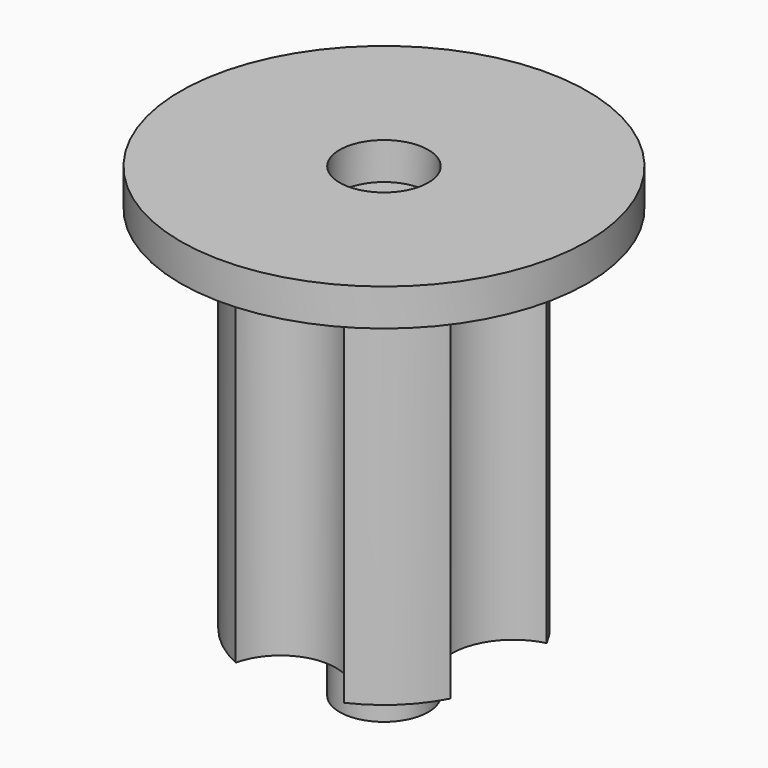
from build123d import *

# Parameters (mm, degrees)
F0_R     = 7.62
F1_DEPTH = 63.5
F0_R_2   = 34.925
F3_DEPTH = 6.35
F4_DEPTH = 73.66


# Not quite as in the source:
# - the program builds the solid bodies; features that only make, move or delete a surface that nothing else refers to are left out


with BuildPart() as f1:
    # F0 (on Top) → F1 (new body)
    with BuildSketch(Plane.XY):
        with BuildLine():
            ThreePointArc((19.6950692857, -10.2982945593), (11.6205, 0), (19.6950692857, 10.2982945593))
            ThreePointArc((19.6950692857, 10.2982945593), (15.0819932796, 16.3243408355), (8.7103855253, 20.447))
            ThreePointArc((8.7103855253, 20.447), (0, 13.335), (-8.7103855253, 20.447))
            ThreePointArc((-8.7103855253, 20.447), (-14.4936529558, 16.8488767874), (-18.9156521429, 11.668278751))
            ThreePointArc((-18.9156521429, 11.668278751), (-12.549310419, 7.3131076419), (-10.0965, 0))
            ThreePointArc((-10.0965, 0), (-12.549310419, -7.3131076419), (-18.9156521429, -11.668278751))
            ThreePointArc((-18.9156521429, -11.668278751), (-14.738135996, -16.6354432572), (-9.3037440003, -20.1839285714))
            ThreePointArc((-9.3037440003, -20.1839285714), (0, -12.7), (9.3037440003, -20.1839285714))
            ThreePointArc((9.3037440003, -20.1839285714), (15.3187542886, -16.102372249), (19.6950692857, -10.2982945593))
        make_face()
        Circle(F0_R, mode=Mode.SUBTRACT)
    extrude(amount=-F1_DEPTH)

    # F0 (on Top) → F3 (join)
    with BuildSketch(Plane.XY):
        Circle(F0_R_2)
        with BuildLine():
            ThreePointArc((8.7103855253, 20.447), (15.0819932796, 16.3243408355), (19.6950692857, 10.2982945593))
            ThreePointArc((19.6950692857, 10.2982945593), (28.7681937917, 8.3451803608), (32.8295, 0))
            ThreePointArc((32.8295, 0), (28.7681937917, -8.3451803608), (19.6950692857, -10.2982945593))
            ThreePointArc((19.6950692857, -10.2982945593), (15.3187542886, -16.102372249), (9.3037440003, -20.1839285714))
            ThreePointArc((9.3037440003, -20.1839285714), (9.4695244496, -21.198485656), (9.525, -22.225))
            ThreePointArc((9.525, -22.225), (-1.026514344, -31.6945244496), (-9.3037440003, -20.1839285714))
            ThreePointArc((-9.3037440003, -20.1839285714), (-14.738135996, -16.6354432572), (-18.9156521429, -11.668278751))
            ThreePointArc((-18.9156521429, -11.668278751), (-34.3535, 0), (-18.9156521429, 11.668278751))
            ThreePointArc((-18.9156521429, 11.668278751), (-14.4936529558, 16.8488767874), (-8.7103855253, 20.447))
            ThreePointArc((-8.7103855253, 20.447), (-0.8935246722, 31.0699824002), (8.89, 22.225))
            ThreePointArc((8.89, 22.225), (8.8449824002, 21.3314753278), (8.7103855253, 20.447))
        make_face(mode=Mode.SUBTRACT)
        with BuildLine():
            ThreePointArc((19.6950692857, -10.2982945593), (11.6205, 0), (19.6950692857, 10.2982945593))
            ThreePointArc((19.6950692857, 10.2982945593), (15.0819932796, 16.3243408355), (8.7103855253, 20.447))
            ThreePointArc((8.7103855253, 20.447), (0, 13.335), (-8.7103855253, 20.447))
            ThreePointArc((-8.7103855253, 20.447), (-14.4936529558, 16.8488767874), (-18.9156521429, 11.668278751))
            ThreePointArc((-18.9156521429, 11.668278751), (-12.549310419, 7.3131076419), (-10.0965, 0))
            ThreePointArc((-10.0965, 0), (-12.549310419, -7.3131076419), (-18.9156521429, -11.668278751))
            ThreePointArc((-18.9156521429, -11.668278751), (-14.738135996, -16.6354432572), (-9.3037440003, -20.1839285714))
            ThreePointArc((-9.3037440003, -20.1839285714), (0, -12.7), (9.3037440003, -20.1839285714))
            ThreePointArc((9.3037440003, -20.1839285714), (15.3187542886, -16.102372249), (19.6950692857, -10.2982945593))
        make_face()
        Circle(F0_R, mode=Mode.SUBTRACT)
        with BuildLine():
            ThreePointArc((-8.7103855253, 20.447), (0, 13.335), (8.7103855253, 20.447))
            ThreePointArc((8.7103855253, 20.447), (0, 22.225), (-8.7103855253, 20.447))
        make_face()
        with BuildLine():
            ThreePointArc((-8.7103855253, 20.447), (0, 22.225), (8.7103855253, 20.447))
            ThreePointArc((8.7103855253, 20.447), (8.8449824002, 21.3314753278), (8.89, 22.225))
            ThreePointArc((8.89, 22.225), (-0.8935246722, 31.0699824002), (-8.7103855253, 20.447))
        make_face()
        with BuildLine():
            ThreePointArc((19.6950692857, -10.2982945593), (21.5832520705, -5.30225), (22.225, 0))
            ThreePointArc((22.225, 0), (21.5832520705, 5.30225), (19.6950692857, 10.2982945593))
            ThreePointArc((19.6950692857, 10.2982945593), (11.6205, 0), (19.6950692857, -10.2982945593))
        make_face()
        with BuildLine():
            ThreePointArc((19.6950692857, 10.2982945593), (21.5832520705, 5.30225), (22.225, 0))
            ThreePointArc((22.225, 0), (21.5832520705, -5.30225), (19.6950692857, -10.2982945593))
            ThreePointArc((19.6950692857, -10.2982945593), (28.7681937917, -8.3451803608), (32.8295, 0))
            ThreePointArc((32.8295, 0), (28.7681937917, 8.3451803608), (19.6950692857, 10.2982945593))
        make_face()
        with BuildLine():
            ThreePointArc((-18.9156521429, -11.668278751), (-22.225, 0), (-18.9156521429, 11.668278751))
            ThreePointArc((-18.9156521429, 11.668278751), (-34.3535, 0), (-18.9156521429, -11.668278751))
        make_face()
        with BuildLine():
            ThreePointArc((-10.0965, 0), (-12.549310419, 7.3131076419), (-18.9156521429, 11.668278751))
            ThreePointArc((-18.9156521429, 11.668278751), (-22.225, 0), (-18.9156521429, -11.668278751))
            ThreePointArc((-18.9156521429, -11.668278751), (-12.549310419, -7.3131076419), (-10.0965, 0))
        make_face()
        with BuildLine():
            ThreePointArc((9.525, -22.225), (9.4695244496, -21.198485656), (9.3037440003, -20.1839285714))
            ThreePointArc((9.3037440003, -20.1839285714), (0, -22.225), (-9.3037440003, -20.1839285714))
            ThreePointArc((-9.3037440003, -20.1839285714), (-1.026514344, -31.6945244496), (9.525, -22.225))
        make_face()
        with BuildLine():
            ThreePointArc((-9.3037440003, -20.1839285714), (0, -22.225), (9.3037440003, -20.1839285714))
            ThreePointArc((9.3037440003, -20.1839285714), (0, -12.7), (-9.3037440003, -20.1839285714))
        make_face()
    extrude(amount=F3_DEPTH)

    # F0 (on Top) → F4 (join)
    with BuildSketch(Plane.XY):
        Circle(F0_R)
    extrude(amount=-F4_DEPTH)


solid = f1.part
